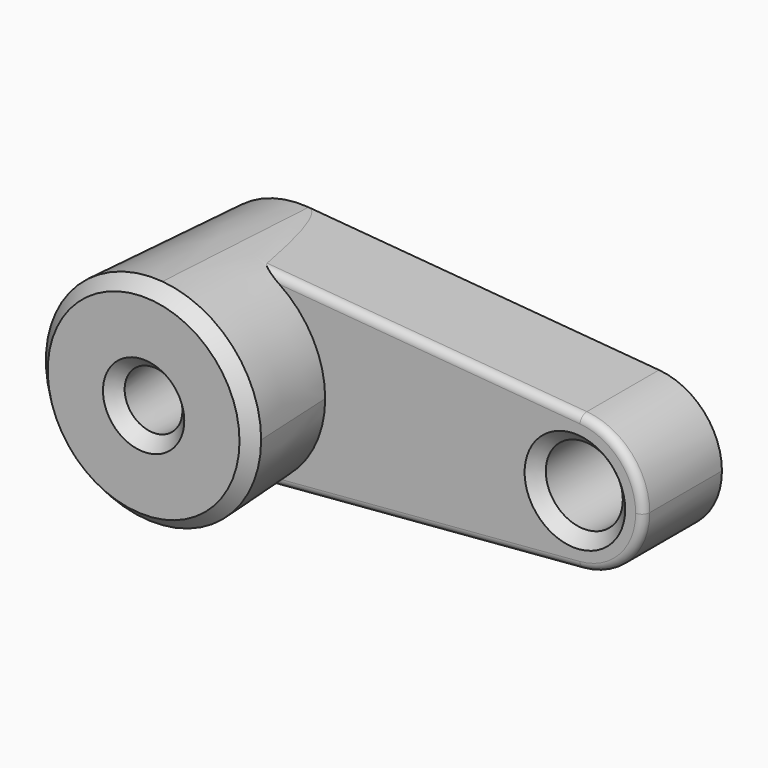
from build123d import *

# Parameters (mm, degrees)
F0_R     = 9.8233576781
F1_DEPTH = 25
F2_DEPTH = 50
F2_TAPER = -3
F4_R     = 2


# Not quite as in the source:
# - a fillet or chamfer that OpenCascade refuses, or shapes differently, is made with other operations: its cross-section is extruded or revolved along the edge and cut away or added


with BuildPart() as f1:
    # F0 (on Front) → F1 (new body)
    with BuildSketch(Plane.XZ):
        with BuildLine():
            ThreePointArc((2.0833333333, 24.9130432148), (18.3995018048, 16.9250800097), (25, 0))
            ThreePointArc((25, 0), (18.3995018048, -16.9250800097), (2.0833333333, -24.9130432148))
            Line((2.0833333333, -24.9130432148), (91.4583333333, -17.4391302504))
            ThreePointArc((91.4583333333, -17.4391302504), (72.5, 0), (91.4583333333, 17.4391302504))
            Line((91.4583333333, 17.4391302504), (2.0833333333, 24.9130432148))
        make_face()
        with BuildLine():
            ThreePointArc((2.0833333333, -24.9130432148), (18.3995018048, -16.9250800097), (25, 0))
            ThreePointArc((25, 0), (18.3995018048, 16.9250800097), (2.0833333333, 24.9130432148))
            ThreePointArc((2.0833333333, 24.9130432148), (-25, 0), (2.0833333333, -24.9130432148))
        make_face()
        Circle(F0_R, mode=Mode.SUBTRACT)
        with BuildLine():
            ThreePointArc((107.5, 0), (102.8796512634, 11.8475560068), (91.4583333333, 17.4391302504))
            ThreePointArc((91.4583333333, 17.4391302504), (72.5, 0), (91.4583333333, -17.4391302504))
            ThreePointArc((91.4583333333, -17.4391302504), (102.8796512634, -11.8475560068), (107.5, 0))
        make_face()
        with Locations((90, 0)):
            Circle(F0_R, mode=Mode.SUBTRACT)
    extrude(amount=F1_DEPTH)

    # F0 (on Front) → F2 (join)
    with BuildSketch(Plane.XZ):
        with BuildLine():
            ThreePointArc((2.0833333333, -24.9130432148), (18.3995018048, -16.9250800097), (25, 0))
            ThreePointArc((25, 0), (18.3995018048, 16.9250800097), (2.0833333333, 24.9130432148))
            ThreePointArc((2.0833333333, 24.9130432148), (-25, 0), (2.0833333333, -24.9130432148))
        make_face()
        Circle(F0_R, mode=Mode.SUBTRACT)
    extrude(amount=F2_DEPTH, taper=F2_TAPER)

    # F3: chamfer of 3 on 3 edges, made by hand

    # F3_s1 → F3_t2 (revolve, cut)
    with BuildSketch(Plane.XY):
        Polygon((102.8233576781, -25), (99.8233576781, -22), (99.8233576781, -25), align=None)
    revolve(axis=Axis((90, -25, 0), (0, -1, 0)), mode=Mode.SUBTRACT)

    # F3_s3 → F3_t4 (revolve, cut)
    with BuildSketch(Plane.XY):
        Polygon((7.3684204855, -46.8429921313), (10.3643090898, -50), (7.2029687139, -50), align=None)
    revolve(axis=Axis((0, -50, 0), (0, 1, 0)), mode=Mode.SUBTRACT)

    # F3_s5 → F3_t6 (revolve, cut)
    with BuildSketch(Plane(origin=(0, 0, 0), x_dir=(0, 1, 0), z_dir=(0.9965217286, 0, 0.0833333333))):
        Polygon((-46.8429921313, -27.4549371926), (-50, -24.4590485883), (-50, -27.6203889642), align=None)
    revolve(axis=Axis((0, -50, 0), (0, 1, 0)), mode=Mode.SUBTRACT)

    # F4
    f4_edges = [f1.edges().sort_by_distance(p)[0] for p in [
        (50.856157, -25, -20.834455),
        (107.5, -25, 0),
        (50.856157, -25, 20.834455),
    ]]
    fillet(f4_edges, radius=F4_R)


solid = f1.part
